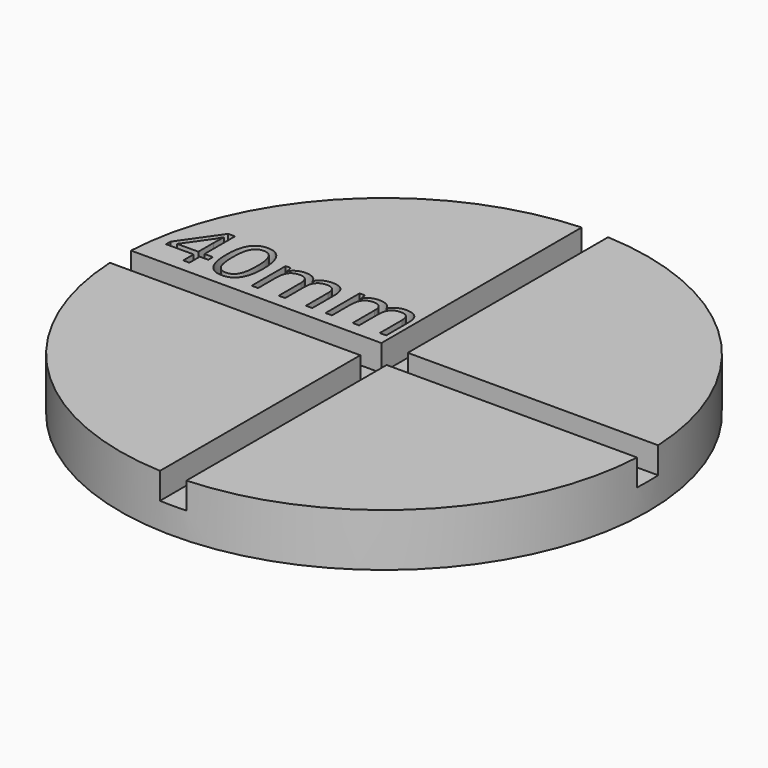
from build123d import *

# Parameters (mm, degrees)
F0_R         = 20
F1_DEPTH     = 4
F2_W         = 24
F2_H         = 2
F2_W_2       = 2
F2_H_2       = 24
F3_DEPTH     = 2
F4_TEXT_SIZE = 6.0214693725
F5_DEPTH     = 1


# Not quite as in the source:
# - Text() gives the source's letters only with a copy of the font that has no kerning and outlines rounded to 1/6400 em; it was checked with that copy


with BuildPart() as f1:
    # F0 (on Top) → F1 (new body)
    with BuildSketch(Plane.XY):
        Circle(F0_R)
    extrude(amount=F1_DEPTH)

    # F2 (on face) → F3 (cut)
    with BuildSketch(Plane.XY.offset(4)):
        with Locations((13, 0)):
            Rectangle(F2_W, F2_H)
        with Locations((0, -13)):
            Rectangle(F2_W_2, F2_H_2)
        Rectangle(F2_W_2, F2_H)
        with Locations((-13, 0)):
            Rectangle(F2_W, F2_H)
        with Locations((0, 13)):
            Rectangle(F2_W_2, F2_H_2)
    extrude(amount=-F3_DEPTH, mode=Mode.SUBTRACT)

    # F4 (on face) → F5 (cut)
    with BuildSketch(Plane.XY.offset(4)):
        with Locations((-18.9891397503, 1.9424853091)):
            Text('40mm', F4_TEXT_SIZE, font='Open Sans', text_align=(TextAlign.LEFT, TextAlign.BOTTOM))
    extrude(amount=-F5_DEPTH, mode=Mode.SUBTRACT)


solid = f1.part
